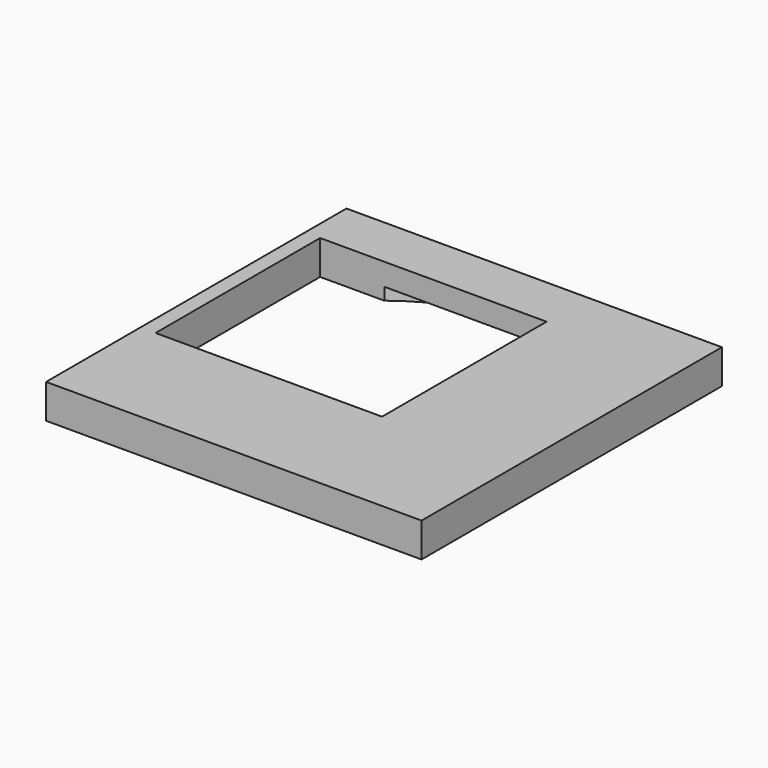
from build123d import *

# Parameters (mm, degrees)
F0_W     = 30.67
F0_H     = 30.67
F1_DEPTH = 1
F0_W_2   = 12.1056904889
F0_H_2   = 1.4927708568
F0_W_3   = 1.4087211761
F0_H_3   = 4.1082873123
F2_DEPTH = 1.8


# Not quite as in the source:
# - a feature names something its author has since deleted; it is built from what else it names


with BuildPart() as f1:
    # F0 (on Top) → F1 (new body)
    with BuildSketch(Plane.XY):
        Rectangle(F0_W, F0_H)
        with BuildLine():
            ThreePointArc((-8.8560749891, 11.0999971075), (6.1596970362, 12.7944570976), (14.2, 0))
            ThreePointArc((14.2, 0), (2.9118804142, -13.8982355878), (-13.0057679512, -5.7))
            Line((-13.0057679512, -5.7), (-14.0999610525, -5.7))
            Line((-14.0999610525, -5.7), (-14.0999610525, -1.6825867938))
            ThreePointArc((-14.0999610525, -1.6825867938), (-14.2, 0), (-14.0999610525, 1.6825867938))
            Line((-14.0999610525, 1.6825867938), (-14.0999610525, 5.7))
            Line((-14.0999610525, 5.7), (-14.0999610525, 11.0999971075))
            Line((-14.0999610525, 11.0999971075), (-8.8560749891, 11.0999971075))
        make_face(mode=Mode.SUBTRACT)
        with BuildLine():
            ThreePointArc((-14.0999610525, 1.6825867938), (-14.2, 0), (-14.0999610525, -1.6825867938))
            Line((-14.0999610525, -1.6825867938), (-14.0999610525, 1.6825867938))
        make_face()
    extrude(amount=-F1_DEPTH)



with BuildPart() as f1b:
    # F0 (on Top) → F1, piece 2 (new body)
    with BuildSketch(Plane.XY):
        with BuildLine():
            Line((2.9913177714, -5.7), (-9.1143727175, -5.7))
            ThreePointArc((-9.1143727175, -5.7), (-3.1266086976, -10.2852600601), (4.4000389475, -9.8082873123))
            ThreePointArc((4.4000389475, -9.8082873123), (10.7500389475, 0), (4.4000389475, 9.8082873123))
            Line((4.4000389475, 9.8082873123), (4.4000389475, 5.7))
            Line((4.4000389475, 5.7), (4.4000389475, 4.2072320357))
            Line((4.4000389475, 4.2072320357), (4.4000389475, -4.2072320357))
            Line((4.4000389475, -4.2072320357), (4.4000389475, -5.7))
            Line((4.4000389475, -5.7), (2.9913177714, -5.7))
        make_face()
        Polygon((2.9913177714, -4.2072291432), (2.9913177714, -5.7), (4.4000389475, -5.7), (4.4000389475, -4.2072320357), (4.4000389475, 4.2072320357), (4.4000389475, 5.7), (2.9913177714, 5.7), (2.9913177714, 4.2072291432), align=None)
        with Locations((-3.0615274731, -4.9536145716)):
            Rectangle(F0_W_2, F0_H_2)
        Polygon((2.9913177714, -4.2072291432), (2.9913177714, -5.7), (4.4000389475, -5.7), (4.4000389475, -4.2072320357), (4.4000389475, 4.2072320357), (4.4000389475, 5.7), (2.9913177714, 5.7), (2.9913177714, 4.2072291432), align=None)
        with Locations((3.6956783594, 7.7541436561)):
            Rectangle(F0_W_3, F0_H_3)
    extrude(amount=-F1_DEPTH)


with BuildPart() as f1_1:
    add(f1.part)

    add(f1b.part)  # F2 merges F1b
    # F0 (on Top) → F2 (join)
    with BuildSketch(Plane.XY):
        Rectangle(F0_W, F0_H)
        with BuildLine():
            ThreePointArc((-8.8560749891, 11.0999971075), (6.1596970362, 12.7944570976), (14.2, 0))
            ThreePointArc((14.2, 0), (2.9118804142, -13.8982355878), (-13.0057679512, -5.7))
            Line((-13.0057679512, -5.7), (-14.0999610525, -5.7))
            Line((-14.0999610525, -5.7), (-14.0999610525, -1.6825867938))
            ThreePointArc((-14.0999610525, -1.6825867938), (-14.2, 0), (-14.0999610525, 1.6825867938))
            Line((-14.0999610525, 1.6825867938), (-14.0999610525, 5.7))
            Line((-14.0999610525, 5.7), (-14.0999610525, 11.0999971075))
            Line((-14.0999610525, 11.0999971075), (-8.8560749891, 11.0999971075))
        make_face(mode=Mode.SUBTRACT)
        with BuildLine():
            ThreePointArc((-13.0057679512, -5.7), (2.9118804142, -13.8982355878), (14.2, 0))
            ThreePointArc((14.2, 0), (6.1596970362, 12.7944570976), (-8.8560749891, 11.0999971075))
            Line((-8.8560749891, 11.0999971075), (2.9913177714, 11.0999971075))
            Line((2.9913177714, 11.0999971075), (4.4000389475, 11.0999971075))
            Line((4.4000389475, 11.0999971075), (4.4000389475, 9.8082873123))
            ThreePointArc((4.4000389475, 9.8082873123), (10.7500389475, 0), (4.4000389475, -9.8082873123))
            ThreePointArc((4.4000389475, -9.8082873123), (-3.1266086976, -10.2852600601), (-9.1143727175, -5.7))
            Line((-9.1143727175, -5.7), (-13.0057679512, -5.7))
        make_face()
        with BuildLine():
            Line((2.9913177714, -5.7), (-9.1143727175, -5.7))
            ThreePointArc((-9.1143727175, -5.7), (-3.1266086976, -10.2852600601), (4.4000389475, -9.8082873123))
            ThreePointArc((4.4000389475, -9.8082873123), (10.7500389475, 0), (4.4000389475, 9.8082873123))
            Line((4.4000389475, 9.8082873123), (4.4000389475, 5.7))
            Line((4.4000389475, 5.7), (4.4000389475, 4.2072320357))
            Line((4.4000389475, 4.2072320357), (4.4000389475, -4.2072320357))
            Line((4.4000389475, -4.2072320357), (4.4000389475, -5.7))
            Line((4.4000389475, -5.7), (2.9913177714, -5.7))
        make_face()
        with BuildLine():
            ThreePointArc((-14.0999610525, 1.6825867938), (-14.2, 0), (-14.0999610525, -1.6825867938))
            Line((-14.0999610525, -1.6825867938), (-14.0999610525, 1.6825867938))
        make_face()
    extrude(amount=F2_DEPTH)


solid = f1_1.part
